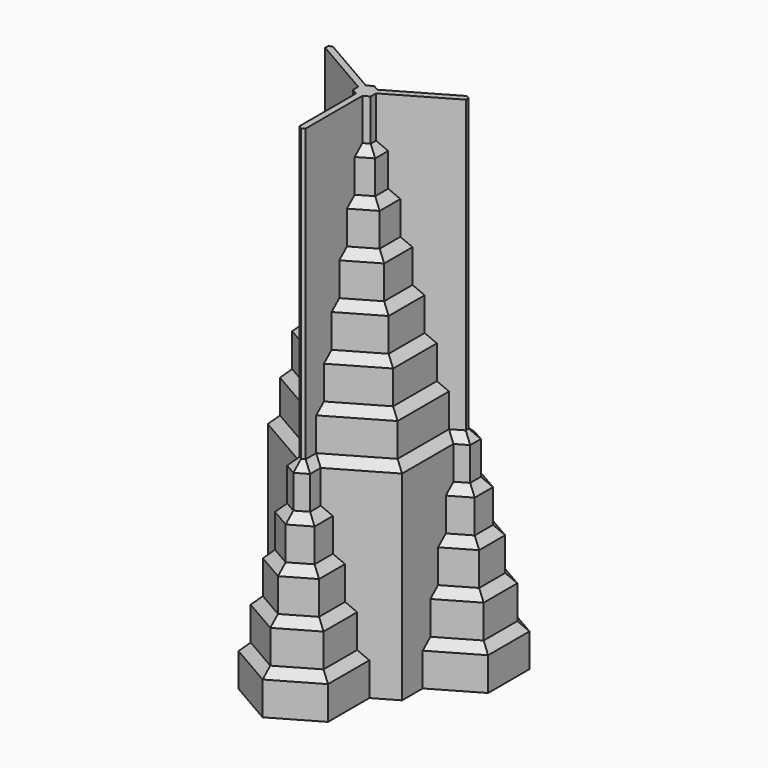
from build123d import *

# Parameters (mm, degrees)
F1_DEPTH  = 25.4
F2_SIZE   = 5.08
F3_DEPTH  = 25.4
F4_SIZE   = 5.08
F5_DEPTH  = 25.4
F6_SIZE   = 5.08
F7_DEPTH  = 25.4
F8_SIZE   = 5.08
F9_DEPTH  = 25.4
F10_SIZE  = 5.08
F12_DEPTH = 25.4
F13_SIZE  = 5.08
F14_DEPTH = 25.4
F15_SIZE  = 5.08
F16_DEPTH = 25.4
F17_SIZE  = 5.08
F18_DEPTH = 25.4
F19_SIZE  = 5.08
F20_DEPTH = 25.4
F21_SIZE  = 5.08
F22_DEPTH = 25.4
F23_SIZE  = 5.08
F24_DEPTH = 25.4


# Not quite as in the source:
# - two fillets or chamfers of one size are made in one step


with BuildPart() as f1:
    # F0 (on Top) → F1 (new body)
    with BuildSketch(Plane.XY):
        Polygon((13.6634483933, 39.4429780398), (40.99034518, 23.6657868239), (40.99034518, -7.888595608), (68.3172419667, 7.888595608), (68.3172419667, 39.4429780398), (40.99034518, 55.2201692557), align=None)
        Polygon((40.99034518, -7.888595608), (40.99034518, 23.6657868239), (13.6634483933, 39.4429780398), (13.6634483933, 7.888595608), align=None)
        Polygon((40.99034518, -23.6657868239), (40.99034518, -7.888595608), (13.6634483933, 7.888595608), (13.6634483933, 39.4429780398), (0, 47.3315736477), (-13.6634483933, 39.4429780398), (-13.6634483933, 7.888595608), (-40.99034518, -7.888595608), (-40.99034518, -23.6657868239), (-27.3268967867, -31.5543824318), (0, -15.7771912159), (27.3268967867, -31.5543824318), align=None)
        Polygon((27.3268967867, -63.1087648636), (27.3268967867, -31.5543824318), (0, -47.3315736477), (-27.3268967867, -31.5543824318), (-27.3268967867, -63.1087648636), (0, -78.8859560796), align=None)
        Polygon((0, -47.3315736477), (27.3268967867, -31.5543824318), (0, -15.7771912159), (-27.3268967867, -31.5543824318), align=None)
        Polygon((-13.6634483933, 7.888595608), (-13.6634483933, 39.4429780398), (-40.99034518, 23.6657868239), (-40.99034518, -7.888595608), align=None)
        Polygon((-40.99034518, 23.6657868239), (-13.6634483933, 39.4429780398), (-40.99034518, 55.2201692557), (-68.3172419667, 39.4429780398), (-68.3172419667, 7.888595608), (-40.99034518, -7.888595608), align=None)
    extrude(amount=F1_DEPTH)

    # F2
    f2_edges = [f1.edges().sort_by_distance(p)[0] for p in [
        (-54.653794, 0, 25.4),
        (-27.326897, -47.331574, 25.4),
        (-13.663448, -70.99736, 25.4),
        (13.663448, -70.99736, 25.4),
        (27.326897, -47.331574, 25.4),
        (54.653794, 0, 25.4),
        (68.317242, 23.665787, 25.4),
        (54.653794, 47.331574, 25.4),
        (27.326897, 47.331574, 25.4),
        (-27.326897, 47.331574, 25.4),
        (-54.653794, 47.331574, 25.4),
        (-68.317242, 23.665787, 25.4),
    ]]
    chamfer(f2_edges, length=F2_SIZE)

    # F3 (add): a face of the model
    f3_faces = [f1.faces().sort_by_distance(p)[0] for p in [
        (0, 0, 25.4),
    ]]
    extrude(f3_faces, amount=F3_DEPTH)

    # F4
    f4_edges = [f1.edges().sort_by_distance(p)[0] for p in [
        (52.113794, 42.932165, 50.8),
        (63.237242, 23.665787, 50.8),
        (52.113794, 4.399409, 50.8),
        (22.246897, -47.331574, 50.8),
        (11.123448, -66.597951, 50.8),
        (-11.123448, -66.597951, 50.8),
        (-22.246897, -47.331574, 50.8),
        (-52.113794, 4.399409, 50.8),
        (-63.237242, 23.665787, 50.8),
        (-52.113794, 42.932165, 50.8),
        (-29.866897, 42.932165, 50.8),
        (29.866897, 42.932165, 50.8),
    ]]
    chamfer(f4_edges, length=F4_SIZE)

    # F5 (add): a face of the model
    f5_faces = [f1.faces().sort_by_distance(p)[0] for p in [
        (0, 0, 50.8),
    ]]
    extrude(f5_faces, amount=F5_DEPTH)

    # F6
    f6_edges = [f1.edges().sort_by_distance(p)[0] for p in [
        (49.573794, 38.532756, 76.2),
        (58.157242, 23.665787, 76.2),
        (49.573794, 8.798818, 76.2),
        (8.583448, -62.198542, 76.2),
        (-8.583448, -62.198542, 76.2),
        (-17.166897, -47.331574, 76.2),
        (-58.157242, 23.665787, 76.2),
        (-49.573794, 38.532756, 76.2),
        (-32.406897, 38.532756, 76.2),
        (-49.573794, 8.798818, 76.2),
        (17.166897, -47.331574, 76.2),
        (32.406897, 38.532756, 76.2),
    ]]
    chamfer(f6_edges, length=F6_SIZE)

    # F7 (add): a face of the model
    f7_faces = [f1.faces().sort_by_distance(p)[0] for p in [
        (0, 0, 76.2),
    ]]
    extrude(f7_faces, amount=F7_DEPTH)

    # F8
    f8_edges = [f1.edges().sort_by_distance(p)[0] for p in [
        (47.033794, 34.133346, 101.6),
        (53.077242, 23.665787, 101.6),
        (47.033794, 13.198227, 101.6),
        (6.043448, -57.799133, 101.6),
        (-6.043448, -57.799133, 101.6),
        (-12.086897, -47.331574, 101.6),
        (-53.077242, 23.665787, 101.6),
        (-47.033794, 34.133346, 101.6),
        (-34.946897, 34.133346, 101.6),
        (-47.033794, 13.198227, 101.6),
        (12.086897, -47.331574, 101.6),
        (34.946897, 34.133346, 101.6),
    ]]
    chamfer(f8_edges, length=F8_SIZE)

    # F9 (add): a face of the model
    f9_faces = [f1.faces().sort_by_distance(p)[0] for p in [
        (0, 0, 101.6),
    ]]
    extrude(f9_faces, amount=F9_DEPTH)

    # F10
    f10_edges = [f1.edges().sort_by_distance(p)[0] for p in [
        (40.990345, -4.045434, 127),
        (23.998621, -33.475963, 127),
        (-23.998621, -33.475963, 127),
        (-40.990345, -4.045434, 127),
        (-16.991724, 37.521397, 127),
        (16.991724, 37.521397, 127),
        (44.493794, 29.733937, 127),
        (47.997242, 23.665787, 127),
        (44.493794, 17.597636, 127),
        (3.503448, -53.399724, 127),
        (-3.503448, -53.399724, 127),
        (-7.006897, -47.331574, 127),
        (-47.997242, 23.665787, 127),
        (-44.493794, 29.733937, 127),
        (-37.486897, 29.733937, 127),
        (-44.493794, 17.597636, 127),
        (7.006897, -47.331574, 127),
        (37.486897, 29.733937, 127),
    ]]
    chamfer(f10_edges, length=F10_SIZE)

    # F12 (add): a face of the model
    f12_faces = [f1.faces().sort_by_distance(p)[0] for p in [
        (0, 0, 127),
    ]]
    extrude(f12_faces, amount=F12_DEPTH)

    # F13
    f13_edges = [f1.edges().sort_by_distance(p)[0] for p in [
        (16.991724, 31.655518, 152.4),
        (-16.991724, 31.655518, 152.4),
        (35.910345, -1.112494, 152.4),
        (18.918621, -30.543024, 152.4),
        (-18.918621, -30.543024, 152.4),
        (-35.910345, -1.112494, 152.4),
    ]]
    chamfer(f13_edges, length=F13_SIZE)

    # F14 (add): a face of the model
    f14_faces = [f1.faces().sort_by_distance(p)[0] for p in [
        (0, 0, 152.4),
    ]]
    extrude(f14_faces, amount=F14_DEPTH)

    # F15
    f15_edges = [f1.edges().sort_by_distance(p)[0] for p in [
        (14.451724, 27.256109, 177.8),
        (-14.451724, 27.256109, 177.8),
        (-30.830345, -1.112494, 177.8),
        (-16.378621, -26.143615, 177.8),
        (16.378621, -26.143615, 177.8),
        (30.830345, -1.112494, 177.8),
    ]]
    chamfer(f15_edges, length=F15_SIZE)

    # F16 (add): a face of the model
    f16_faces = [f1.faces().sort_by_distance(p)[0] for p in [
        (0, 0, 177.8),
    ]]
    extrude(f16_faces, amount=F16_DEPTH)

    # F17
    f17_edges = [f1.edges().sort_by_distance(p)[0] for p in [
        (-11.911724, 22.8567, 203.2),
        (-25.750345, -1.112494, 203.2),
        (-13.838621, -21.744206, 203.2),
        (13.838621, -21.744206, 203.2),
        (25.750345, -1.112494, 203.2),
        (11.911724, 22.8567, 203.2),
    ]]
    chamfer(f17_edges, length=F17_SIZE)

    # F18 (add): a face of the model
    f18_faces = [f1.faces().sort_by_distance(p)[0] for p in [
        (0, 0, 203.2),
    ]]
    extrude(f18_faces, amount=F18_DEPTH)

    # F19
    f19_edges = [f1.edges().sort_by_distance(p)[0] for p in [
        (-9.371724, 18.457291, 228.6),
        (-20.670345, -1.112494, 228.6),
        (-11.298621, -17.344797, 228.6),
        (11.298621, -17.344797, 228.6),
        (20.670345, -1.112494, 228.6),
        (9.371724, 18.457291, 228.6),
    ]]
    chamfer(f19_edges, length=F19_SIZE)

    # F20 (add): a face of the model
    f20_faces = [f1.faces().sort_by_distance(p)[0] for p in [
        (0, 0, 228.6),
    ]]
    extrude(f20_faces, amount=F20_DEPTH)

    # F21
    f21_edges = [f1.edges().sort_by_distance(p)[0] for p in [
        (-6.831724, 14.057882, 254),
        (-15.590345, -1.112494, 254),
        (-8.758621, -12.945388, 254),
        (8.758621, -12.945388, 254),
        (15.590345, -1.112494, 254),
        (6.831724, 14.057882, 254),
    ]]
    chamfer(f21_edges, length=F21_SIZE)

    # F22 (add): a face of the model
    f22_faces = [f1.faces().sort_by_distance(p)[0] for p in [
        (0, 0, 254),
    ]]
    extrude(f22_faces, amount=F22_DEPTH)

    # F23
    f23_edges = [f1.edges().sort_by_distance(p)[0] for p in [
        (-4.291724, 9.658473, 279.4),
        (-10.510345, -1.112494, 279.4),
        (-6.218621, -8.545979, 279.4),
        (6.218621, -8.545979, 279.4),
        (10.510345, -1.112494, 279.4),
        (4.291724, 9.658473, 279.4),
    ]]
    chamfer(f23_edges, length=F23_SIZE)

    # F24 (add): a face of the model
    f24_faces = [f1.faces().sort_by_distance(p)[0] for p in [
        (0, 0, 279.4),
    ]]
    extrude(f24_faces, amount=F24_DEPTH)


solid = f1.part
